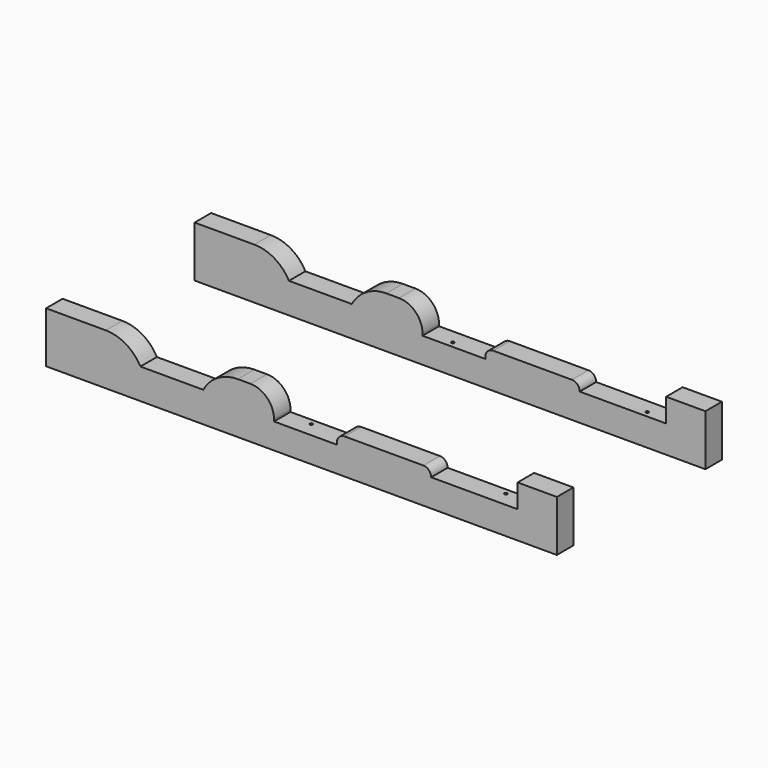
from build123d import *

# Parameters (mm, degrees)
F1_DEPTH     = 66.675
F2_R         = 4.7625
F3_DEPTH     = 12.7
F4_R         = 4.7625
F5_DEPTH     = 12.7
F6_R         = 76.2
F7_R         = 25.39999
F10_W        = 203.2
F10_H        = 66.675
F11_DEPTH    = 66.676
F12_T1_DEPTH = 625.4659800408


# Not quite as in the source:
# - a fillet or chamfer that OpenCascade refuses, or shapes differently, is made with other operations: its cross-section is extruded or revolved along the edge and cut away or added
# - a fillet or chamfer is up to 0.001 mm smaller than in the source, because OpenCascade refuses the exact size


with BuildPart() as f1:
    # F0 (on Front) → F1 (new body)
    with BuildSketch(Plane.XZ):
        Polygon((0, 165.1), (0, 0), (1651, 0), (1651, 165.1), (1524, 165.1), (1524, 88.9), (1244.6, 88.9), (1244.6, 114.3), (939.8, 114.3), (939.8, 82.55), (736.6, 82.55), (736.6, 165.1), align=None)
    extrude(amount=-F1_DEPTH)

    # F2 (on face) → F3 (cut)
    with BuildSketch(Plane.XY.offset(82.55)):
        with Locations((819.15, 19.05)):
            Circle(F2_R)
    extrude(amount=-F3_DEPTH, mode=Mode.SUBTRACT)

    # F4 (on face) → F5 (cut)
    with BuildSketch(Plane.XY.offset(88.9)):
        with Locations((1447.8, 19.05)):
            Circle(F4_R)
    extrude(amount=-F5_DEPTH, mode=Mode.SUBTRACT)

    # F6
    f6_edges = [f1.edges().sort_by_distance(p)[0] for p in [
        (736.6, 33.3375, 165.1),
    ]]
    fillet(f6_edges, radius=F6_R)

    # F7 (radius 25.4 in the source; OpenCascade refuses exactly that, so slightly less here)
    f7_edges = [f1.edges().sort_by_distance(p)[0] for p in [
        (939.8, 33.3375, 114.3),
        (1244.6, 33.3375, 114.3),
    ]]
    fillet(f7_edges, radius=F7_R)


with BuildPart() as f9_1:
    # F9: instance of F1
    add(f1.part.mirror(Plane(origin=(751.1055710536, -266.7, 70.5390726634), x_dir=(1, 0, 0), z_dir=(0, -1, 0))))


with BuildPart() as f1_1:
    add(f1.part)

    # F10 (on face) → F11 (cut, through all)
    with BuildSketch(Plane.XZ):
        with Locations((406.4, 131.7625)):
            Rectangle(F10_W, F10_H)
    extrude(amount=-F11_DEPTH, mode=Mode.SUBTRACT)

    # F12: fillet of radius 127 on 2 edges, made by hand

    # F12_s2 → F12_t1 (cut)
    with BuildSketch(Plane.XZ.offset(-346.0704900204)):
        with BuildLine():
            ThreePointArc((193.0418039918, 165.1), (258.1099413557, 147.164831637), (304.8, 98.425))
            Line((304.8, 98.425), (304.8, 165.1))
            Line((304.8, 165.1), (193.0418039918, 165.1))
        make_face()
        with BuildLine():
            ThreePointArc((508, 98.425), (554.6900586443, 147.164831637), (619.7581960082, 165.1))
            Line((619.7581960082, 165.1), (508, 165.1))
            Line((508, 165.1), (508, 98.425))
        make_face()
    extrude(amount=F12_T1_DEPTH, mode=Mode.SUBTRACT)


with BuildPart() as f14_1:
    # F14: instance of F1
    add(f1_1.part.mirror(Plane(origin=(751.1055710536, -266.7, 70.5390726634), x_dir=(1, 0, 0), z_dir=(0, -1, 0))))


with BuildPart() as f16_1:
    # F16: instance of F1
    add(f1_1.part.mirror(Plane(origin=(751.1055710536, -266.7, 70.5390726634), x_dir=(1, 0, 0), z_dir=(0, -1, 0))))


solid = Compound([f1_1.part, f16_1.part])
